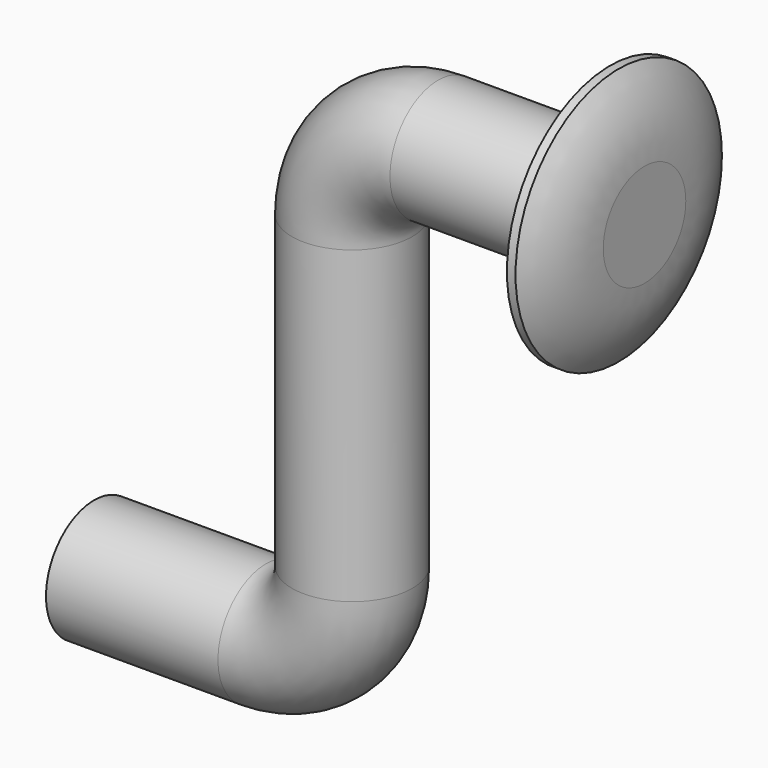
from build123d import *

# Parameters (mm, degrees)
F1_R     = 3.5
F3_R     = 7.5
F3_R_2   = 3.5
F4_DEPTH = 0.5
F5_DEPTH = 0.5
F6_DEPTH = 1.5


# Not quite as in the source:
# - a fillet or chamfer that OpenCascade refuses, or shapes differently, is made with other operations: its cross-section is extruded or revolved along the edge and cut away or added
# - a feature names something its author has since deleted; it is built from what else it names


with BuildPart() as f2:
    # F2: sweep along a path in F0
    with BuildLine(Plane.XZ) as f2_path:
        Line((0, 0), (10, 0))
        ThreePointArc((10, 0), (13.5355339059, 1.4644660941), (15, 5))
        Line((15, 5), (15, 23))
        ThreePointArc((15, 23), (16.4644660941, 26.5355339059), (20, 28))
        Line((20, 28), (30, 28))
    # F1 (on Right) → F2 (sweep)
    with BuildSketch(Plane.YZ):
        Circle(F1_R)
    sweep(path=f2_path.line)

    # F3 (on face) → F4 (join)
    with BuildSketch(Plane.YZ.offset(30)):
        with Locations((0, 28)):
            Circle(F3_R)
        with Locations((0, 28)):
            Circle(F3_R_2, mode=Mode.SUBTRACT)
    extrude(amount=F4_DEPTH)

    # F5 (add): a face of the model
    f5_faces = [f2.faces().sort_by_distance(p)[0] for p in [
        (30, 0, 28),
    ]]
    extrude(f5_faces, amount=F5_DEPTH)


with BuildPart() as f6:
    # F6 (new): a face of the model
    f6_faces = [f2.part.faces().sort_by_distance(p)[0] for p in [
        (30.5, 0, 28),
    ]]
    extrude(f6_faces, amount=F6_DEPTH)

    # F7: fillet of radius 7.5 on 1 edges, made by hand

    # F7_s1 → F7_t2 (revolve, cut)
    with BuildSketch(Plane.XY.offset(28)):
        with BuildLine():
            ThreePointArc((30.5, 7.5), (31.6151247354, 5.3717082451), (32, 3))
            Line((32, 3), (32, 7.5))
            Line((32, 7.5), (30.5, 7.5))
        make_face()
    revolve(axis=Axis((32, 0, 28), (1, 0, 0)), mode=Mode.SUBTRACT)


solid = Compound([f2.part, f6.part])
